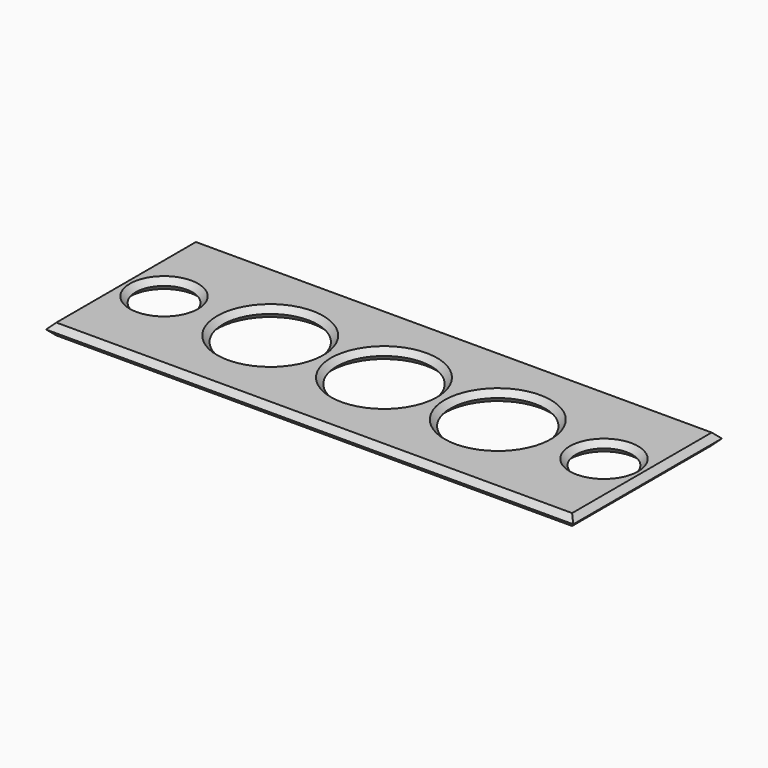
from build123d import *

# Parameters (mm, degrees)
F0_W        = 70
F0_H        = 25
F1_DEPTH    = 1.5
F2_D        = 7
F3_D        = 12
F4_SIZE     = 1
F5_T1_DEPTH = 75.1433659759
F5_T3_DEPTH = 30.1433659759


# Not quite as in the source:
# - a fillet or chamfer that OpenCascade refuses, or shapes differently, is made with other operations: its cross-section is extruded or revolved along the edge and cut away or added


with BuildPart() as f1:
    # F0 (on Top) → F1 (new body)
    with BuildSketch(Plane.XY):
        Rectangle(F0_W, F0_H)
    extrude(amount=F1_DEPTH)

    # F2 (through all)
    with Locations(Plane(origin=(0, 0, 0), x_dir=(1, 0, 0), z_dir=(0, 0, -1))):
        with Locations((-29, 0), (29, 0)):
            Hole(F2_D / 2)

    # F3 (through all)
    with Locations(Plane(origin=(0, 0, 0), x_dir=(1, 0, 0), z_dir=(0, 0, -1))):
        with Locations((-15, 0), (0, 0), (15, 0)):
            Hole(F3_D / 2)

    # F4
    f4_edges = [f1.edges().sort_by_distance(p)[0] for p in [
        (0, -12.5, 1.5),
        (-35, 0, 1.5),
        (35, 0, 1.5),
        (0, 12.5, 1.5),
        (-32.5, 0, 1.5),
        (-21, 0, 1.5),
        (-6, 0, 1.5),
        (9, 0, 1.5),
        (25.5, 0, 1.5),
    ]]
    chamfer(f4_edges, length=F4_SIZE)

    # F5: chamfer of 1 on 9 edges, made by hand

    # F5_s2 → F5_t1 (cut)
    with BuildSketch(Plane.YZ.offset(-37.571682988)):
        Polygon((-12.5, 1), (-11.5, 0), (-12.5, 0), align=None)
        Polygon((11.5, 0), (12.5, 1), (12.5, 0), align=None)
    extrude(amount=F5_T1_DEPTH, mode=Mode.SUBTRACT)

    # F5_s4 → F5_t3 (cut)
    with BuildSketch(Plane.XZ.offset(-15.071682988)):
        Polygon((-35, 1), (-34, 0), (-35, 0), align=None)
        Polygon((34, 0), (35, 1), (35, 0), align=None)
    extrude(amount=F5_T3_DEPTH, mode=Mode.SUBTRACT)

    # F5_s5 → F5_t6 (revolve, cut)
    with BuildSketch(Plane.XZ):
        Polygon((-24.5, 0), (-25.5, 1), (-25.5, 0), align=None)
    revolve(axis=Axis((-29, 0, 0), (0, 0, -1)), mode=Mode.SUBTRACT)

    # F5_s7 → F5_t8 (revolve, cut)
    with BuildSketch(Plane.XZ):
        Polygon((-8, 0), (-9, 1), (-9, 0), align=None)
    revolve(axis=Axis((-15, 0, 0), (0, 0, -1)), mode=Mode.SUBTRACT)

    # F5_s9 → F5_t10 (revolve, cut)
    with BuildSketch(Plane.XZ):
        Polygon((7, 0), (6, 1), (6, 0), align=None)
    revolve(axis=Axis((0, 0, 0), (0, 0, -1)), mode=Mode.SUBTRACT)

    # F5_s11 → F5_t12 (revolve, cut)
    with BuildSketch(Plane.XZ):
        Polygon((22, 0), (21, 1), (21, 0), align=None)
    revolve(axis=Axis((15, 0, 0), (0, 0, -1)), mode=Mode.SUBTRACT)

    # F5_s13 → F5_t14 (revolve, cut)
    with BuildSketch(Plane.XZ):
        Polygon((33.5, 0), (32.5, 1), (32.5, 0), align=None)
    revolve(axis=Axis((29, 0, 0), (0, 0, -1)), mode=Mode.SUBTRACT)


solid = f1.part
